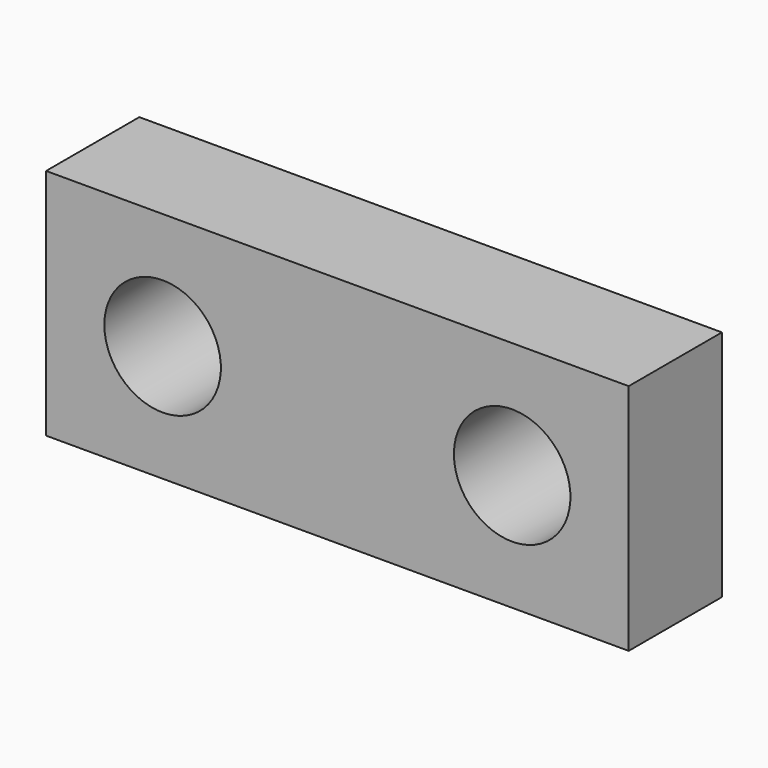
from build123d import *

# Parameters (mm, degrees)
F0_W     = 63.5
F0_H     = 25.4
F1_DEPTH = 12.7
F3_D     = 12.7


# Not quite as in the source:
# - a length typed as a fraction of an inch, garbled in the dataset ("3 / 203.2 mm" for 3/8 in), is restored


with BuildPart() as f1:
    # F0 (on Front) → F1 (new body)
    with BuildSketch(Plane.XZ):
        Rectangle(F0_W, F0_H)
    extrude(amount=F1_DEPTH)

    # F3 (through all)
    with Locations(Plane.XZ.offset(12.7)):
        with Locations((-19.05, 0), (19.05, 0)):
            Hole(F3_D / 2)


solid = f1.part
